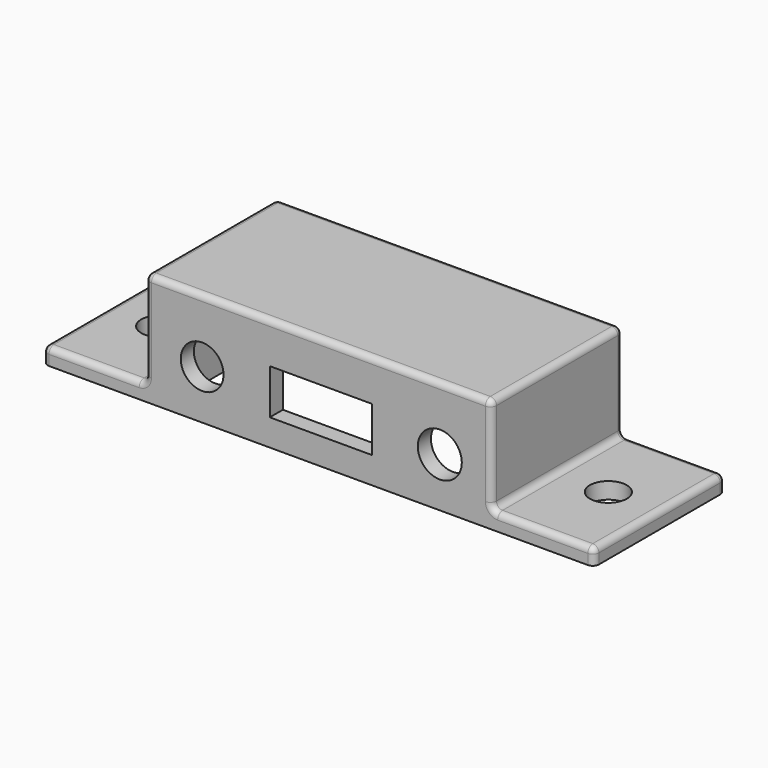
from build123d import *

# Parameters (mm, degrees)
F1_DEPTH = 10.16
F3_D     = 2.286
F4_W     = 19.431
F4_H     = 5.969
F4_R     = 1.3254329065
F4_W_2   = 6.35
F4_H_2   = 2.794
F4_R_2   = 1.3633247541
F5_DEPTH = 1.016
F6_R     = 0.381


with BuildPart() as f1:
    # F0 (on Front) → F1 (new body)
    with BuildSketch(Plane.XZ):
        Polygon((-7.366, 1.016), (-7.366, 0), (0, 0), (0, 5.969), (19.431, 5.969), (19.431, 0), (26.797, 0), (26.797, 1.016), (20.447, 1.016), (20.447, 6.985), (-1.016, 6.985), (-1.016, 1.016), align=None)
    extrude(amount=F1_DEPTH)

    # F3 (through all)
    with Locations(Plane.XY.offset(1.016)):
        with Locations((-4.191, -5.08), (23.622, -5.08)):
            Hole(F3_D / 2)

    # F4 (on face) → F5 (join)
    with BuildSketch(Plane.XZ.offset(10.16)):
        with Locations((9.7155, 2.9845)):
            Rectangle(F4_W, F4_H)
        with Locations((2.5069266703, 3.048)):
            Circle(F4_R, mode=Mode.SUBTRACT)
        with Locations((9.8729266703, 3.048)):
            Rectangle(F4_W_2, F4_H_2, mode=Mode.SUBTRACT)
        with Locations((17.2389266703, 3.0497561675)):
            Circle(F4_R_2, mode=Mode.SUBTRACT)
    extrude(amount=-F5_DEPTH)

    # F6
    f6_edges = [f1.edges().sort_by_distance(p)[0] for p in [
        (20.447, -5.08, 6.985),
        (-1.016, -5.08, 6.985),
        (9.7155, 0, 6.985),
        (9.7155, -10.16, 6.985),
        (-1.016, -10.16, 4.0005),
        (-1.016, -5.08, 1.016),
        (-4.191, -10.16, 1.016),
        (-7.366, -10.16, 0.508),
        (-7.366, -5.08, 1.016),
        (-7.366, 0, 0.508),
        (-4.191, 0, 1.016),
        (0, 0, 2.9845),
        (9.7155, 0, 5.969),
        (19.431, 0, 2.9845),
        (20.447, 0, 4.0005),
        (20.447, -5.08, 1.016),
        (23.622, 0, 1.016),
        (26.797, 0, 0.508),
        (26.797, -5.08, 1.016),
        (26.797, -10.16, 0.508),
        (23.622, -10.16, 1.016),
        (20.447, -10.16, 4.0005),
        (-1.016, 0, 4.0005),
    ]]
    fillet(f6_edges, radius=F6_R)


solid = f1.part
